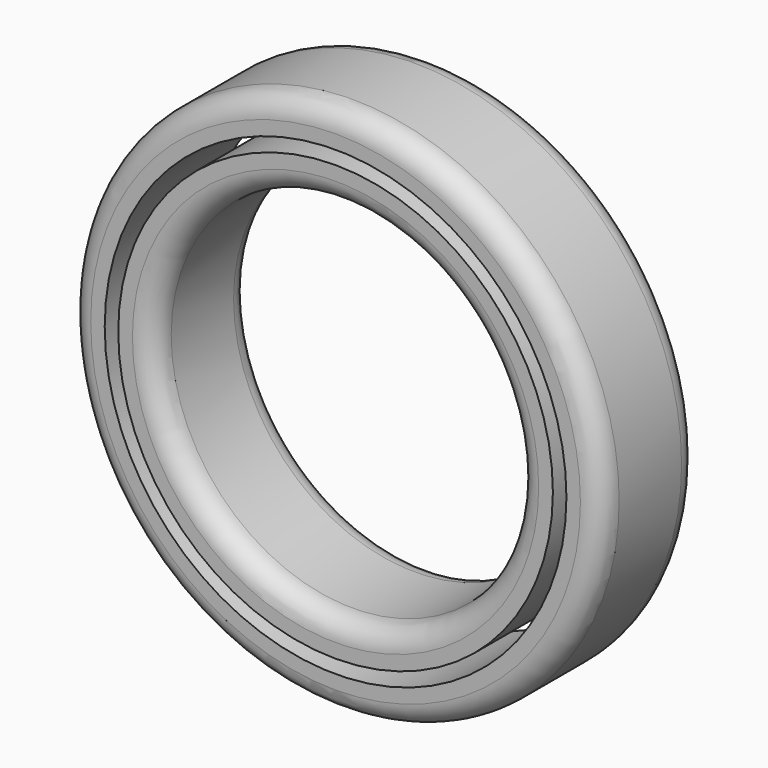
from build123d import *

# Parameters (mm, degrees)
F0_R     = 110
F1_DEPTH = 50
F2_R     = 75
F3_DEPTH = 50.001
F7_R     = 8.89
F8_R     = 95.3337412029
F8_R_2   = 89.742282657
F9_DEPTH = 50.001


# Not quite as in the source:
# - the program builds the solid bodies; features that only make, move or delete a surface that nothing else refers to are left out


with BuildPart() as f1:
    # F0 (on Front) → F1 (new body)
    with BuildSketch(Plane.XZ):
        Circle(F0_R)
    extrude(amount=F1_DEPTH)

    # F2 (on face) → F3 (cut, through all)
    with BuildSketch(Plane.XZ.offset(50)):
        Circle(F2_R)
    extrude(amount=-F3_DEPTH, mode=Mode.SUBTRACT)

    # F7
    f7_edges = [f1.edges().sort_by_distance(p)[0] for p in [
        (-110, -50, 0),
        (-75, -50, 0),
        (-110, 0, 0),
        (-75, 0, 0),
    ]]
    fillet(f7_edges, radius=F7_R)

    # F8 (on face) → F9 (cut, through all)
    with BuildSketch(Plane.XZ.offset(50)):
        Circle(F8_R)
        Circle(F8_R_2, mode=Mode.SUBTRACT)
    extrude(amount=-F9_DEPTH, mode=Mode.SUBTRACT)


solid = f1.part
